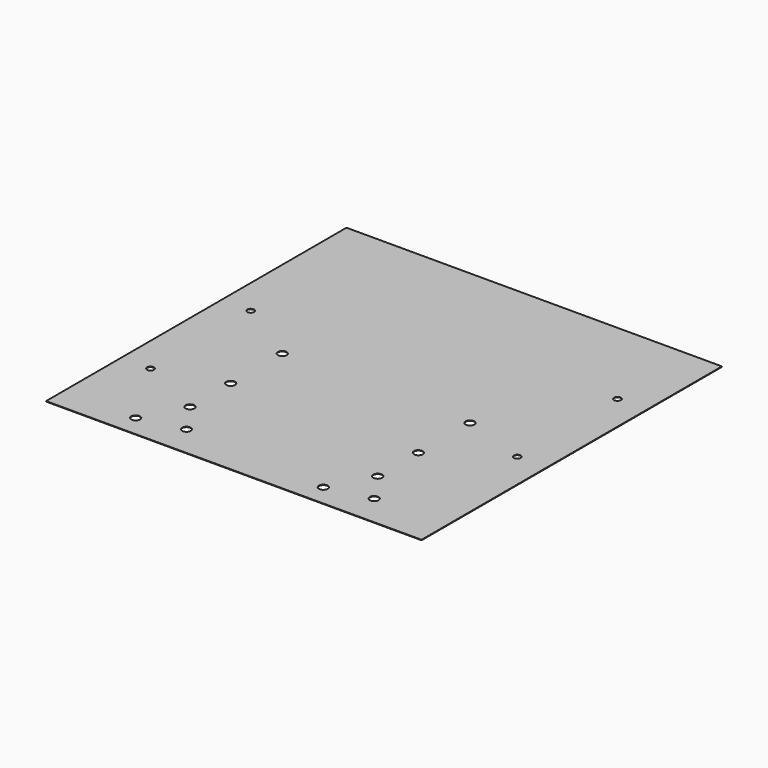
from build123d import *

# Parameters (mm, degrees)
F0_W     = 609.6
F0_H     = 609.6
F1_DEPTH = 0.79375
F2_R     = 5.55625
F3_DEPTH = 25.4
F4_R     = 7.14375
F5_DEPTH = 25.4


# Not quite as in the source:
# - a feature names something its author has since deleted; it is built from what else it names


with BuildPart() as f1:
    # F0 (on Top) → F1 (new body)
    with BuildSketch(Plane.XY):
        with Locations((304.8, 304.8)):
            Rectangle(F0_W, F0_H)
    extrude(amount=F1_DEPTH)

    # F2 (on face) → F3 (cut)
    with BuildSketch(Plane.XY.offset(0.79375)):
        with Locations((47.625, 152.4)):
            Circle(F2_R)
        with Locations((47.625, 355.6)):
            Circle(F2_R)
        with Locations((561.975, 254)):
            Circle(F2_R)
        with Locations((561.975, 457.2)):
            Circle(F2_R)
    extrude(amount=-F3_DEPTH, mode=Mode.SUBTRACT)

    # F4 (on face) → F5 (cut)
    with BuildSketch(Plane.XY.offset(0.79375)):
        with Locations((187.325, 50.8)):
            Circle(F4_R)
        with Locations((117.475, 34.925)):
            Circle(F4_R)
        with Locations((152.4, 101.6)):
            Circle(F4_R)
        with Locations((152.4, 184.15)):
            Circle(F4_R)
        with Locations((152.4, 288.925)):
            Circle(F4_R)
        with Locations((422.275, 34.925)):
            Circle(F4_R)
        with Locations((492.125, 50.8)):
            Circle(F4_R)
        with Locations((457.2, 101.6)):
            Circle(F4_R)
        with Locations((457.2, 184.15)):
            Circle(F4_R)
        with Locations((457.2, 288.925)):
            Circle(F4_R)
    extrude(amount=-F5_DEPTH, mode=Mode.SUBTRACT)


solid = f1.part
